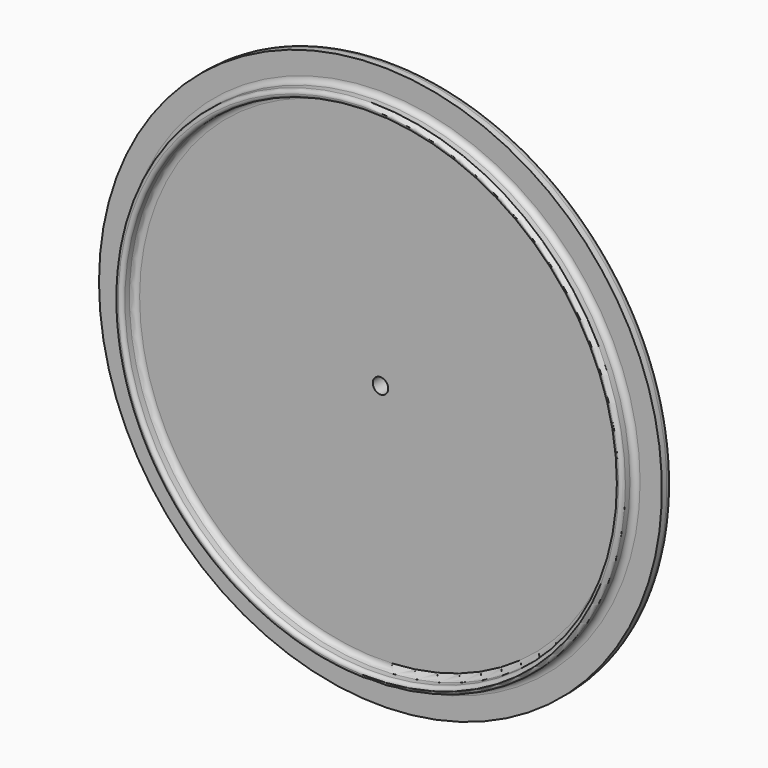
from build123d import *

# Parameters (mm, degrees)
F2_R     = 67.5
F2_R_2   = 65.5
F3_DEPTH = 4
F4_R     = 0.99999
F5_R     = 1.5
F6_R     = 2
F7_R     = 2.05
F8_DEPTH = 6.2575644614


# Not quite as in the source:
# - a fillet or chamfer is up to 0.001 mm smaller than in the source, because OpenCascade refuses the exact size


with BuildPart() as f1:
    # F0 (on Top) → F1 (revolve)
    with BuildSketch(Plane.XY):
        with BuildLine():
            add(Edge.make_bspline(
                [(-74.796, 0), (-63.2667945233, 0.9578141715), (-36.2383694529, 2.7601661408), (-11.99670654, 2.7739654731), (0, 2.7481611414)],
                knots=[0, 0, 0, 0, 0.5050477324, 1, 1, 1, 1], degree=3))
            Line((-74.796, 0), (-74.796, -3.5))
            Line((-74.796, -3.5), (0, -3.5))
            Line((0, -3.5), (0, 0))
            Line((0, 0), (0, 2.7481611414))
        make_face()
    revolve(axis=Axis((0, -1.75, 0), (0, 1, 0)))

    # F2 (on face) → F3 (join)
    with BuildSketch(Plane.XZ.offset(3.5)):
        Circle(F2_R)
        Circle(F2_R_2, mode=Mode.SUBTRACT)
    extrude(amount=F3_DEPTH)

    # F4 (radius 1 in the source; OpenCascade refuses exactly that, so slightly less here)
    f4_edges = [f1.edges().sort_by_distance(p)[0] for p in [
        (-65.5, -7.5, 0),
        (-67.5, -7.5, 0),
    ]]
    fillet(f4_edges, radius=F4_R)

    # F5
    f5_edges = [f1.edges().sort_by_distance(p)[0] for p in [
        (-65.5, -3.5, 0),
        (-67.5, -3.5, 0),
    ]]
    fillet(f5_edges, radius=F5_R)

    # F6
    f6_edges = [f1.edges().sort_by_distance(p)[0] for p in [
        (74.796, 0, 0),
    ]]
    fillet(f6_edges, radius=F6_R)

    # F7 (on face) → F8 (cut, through all)
    with BuildSketch(Plane.XZ.offset(3.5)):
        Circle(F7_R)
    extrude(amount=-F8_DEPTH, mode=Mode.SUBTRACT)


solid = f1.part
